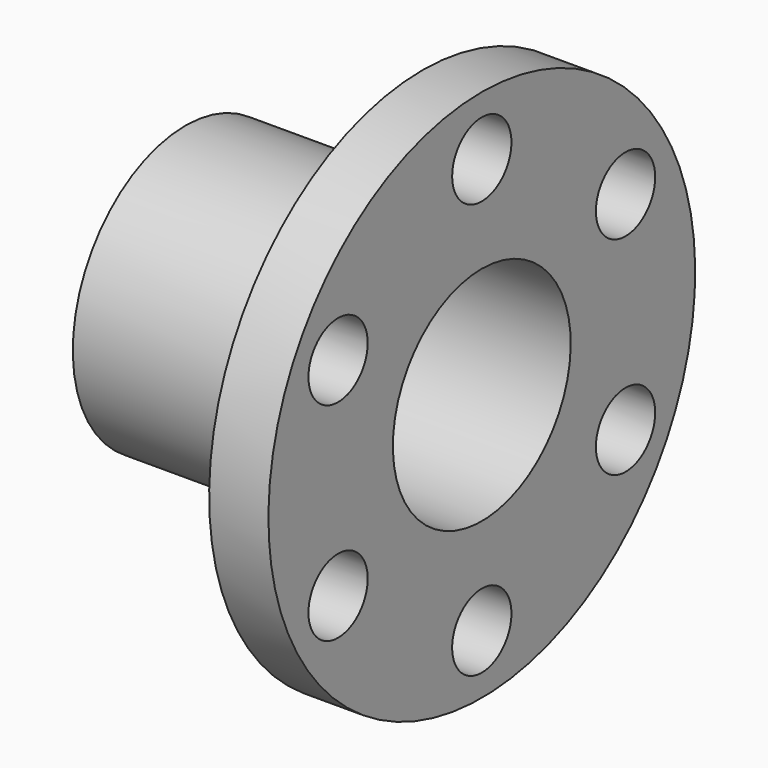
from build123d import *

# Parameters (mm, degrees)
F2_R            = 12.5
F3_DEPTH        = 20.001
F3_COPIES_COUNT = 6


# Not quite as in the source:
# - a pattern or mirror of a feature is missing from the dataset's text; its kind, count and spacing are read off the source's solid


with BuildPart() as f1:
    # F0 (on Front) → F1 (revolve)
    with BuildSketch(Plane.XZ):
        Polygon((-100, 37.5), (0, 37.5), (0, 90), (-20, 90), (-20, 47.5), (-100, 47.5), align=None)
    revolve(axis=Axis((-107.4553492388, 0, 0), (-1, 0, 0)))

    # F2 (on face) → F3 (cut, through all)
    with BuildSketch(Plane(origin=(-20, 0, 0), x_dir=(0, -1, 0), z_dir=(-1, 0, 0))):
        with Locations((0, 70)):
            Circle(F2_R)
    f3 = extrude(amount=-F3_DEPTH, mode=Mode.SUBTRACT)

    # F3_copies: F3 ×6 about axis
    f3_copies_axis = Axis((0, 0, 0), (1, 0, 0))
    for i in range(1, F3_COPIES_COUNT):
        add(f3.rotate(f3_copies_axis, i * 360 / F3_COPIES_COUNT), mode=Mode.SUBTRACT)


solid = f1.part
